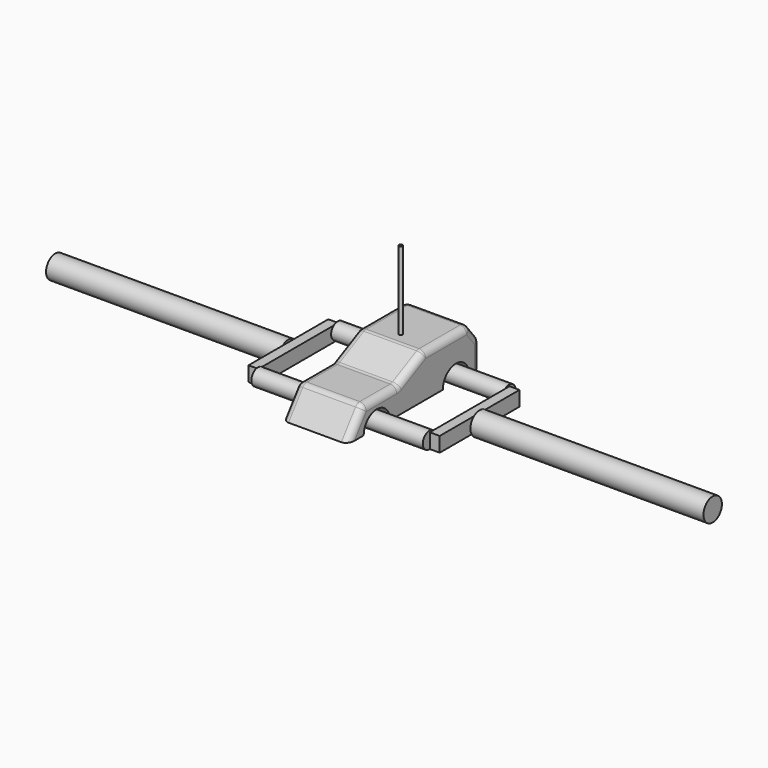
from build123d import *

# Parameters (mm, degrees)
F1_DEPTH  = 25.4
F2_R      = 5.08
F4_DEPTH  = 10.16
F6_DEPTH  = 10.16
F7_R      = 6.35
F8_DEPTH  = 50.8
F10_W     = 76.8076643543
F10_H     = 11.4133090087
F11_DEPTH = 7.62
F13_R     = 8.89
F14_DEPTH = 179.578
F16_R     = 1.27
F17_DEPTH = 60.198


# Not quite as in the source:
# - a feature names something its author has since deleted; it is built from what else it names


with BuildPart() as f1:
    # F0 (on Right) → F1 (new body, symmetric)
    with BuildSketch(Plane.YZ):
        Polygon((-60.8564667081, 20.32), (-76.0964667081, 0), (50.9035332919, 0), (50.9035332919, 20.32), (40.7435332919, 33.02), (-2.4364667081, 33.02), (-27.8364667081, 20.32), align=None)
    extrude(amount=F1_DEPTH, both=True)

    # F2
    f2_edges = [f1.edges().sort_by_distance(p)[0] for p in [
        (25.4, -68.476467, 10.16),
        (25.4, -44.346467, 20.32),
        (25.4, -15.136467, 26.67),
        (25.4, 19.153533, 33.02),
        (25.4, 45.823533, 26.67),
        (25.4, 50.903533, 10.16),
        (0, 50.903533, 20.32),
        (0, 40.743533, 33.02),
        (0, -60.856467, 20.32),
        (0, -27.836467, 20.32),
        (0, -2.436467, 33.02),
        (-25.4, -15.136467, 26.67),
        (-25.4, -44.346467, 20.32),
        (-25.4, -68.476467, 10.16),
        (-25.4, 19.153533, 33.02),
        (-25.4, 50.903533, 10.16),
        (-25.4, 45.823533, 26.67),
    ]]
    fillet(f2_edges, radius=F2_R)

    # F3 (on face) → F4 (cut)
    with BuildSketch(Plane.YZ.offset(25.4)):
        with BuildLine():
            Line((-60.8564667081, 0), (-35.4564667081, 0))
            ThreePointArc((-35.4564667081, 0), (-48.1564667081, 12.7), (-60.8564667081, 0))
        make_face()
        with BuildLine():
            ThreePointArc((40.7435332919, 0), (28.0435332919, 12.7), (15.3435332919, 0))
            Line((15.3435332919, 0), (40.7435332919, 0))
        make_face()
    extrude(amount=-F4_DEPTH, mode=Mode.SUBTRACT)

    # F5 (on face) → F6 (cut)
    with BuildSketch(Plane(origin=(-25.4, 0, 0), x_dir=(0, -1, 0), z_dir=(-1, 0, 0))):
        with BuildLine():
            Line((-40.7435332919, 0), (-15.3435332919, 0))
            ThreePointArc((-15.3435332919, 0), (-28.0435332919, 12.7), (-40.7435332919, 0))
        make_face()
        with BuildLine():
            Line((35.4564667081, 0), (60.8564667081, 0))
            ThreePointArc((60.8564667081, 0), (48.1564667081, 12.7), (35.4564667081, 0))
        make_face()
    extrude(amount=-F6_DEPTH, mode=Mode.SUBTRACT)

    # F7 (on face) → F8 (join)
    with BuildSketch(Plane.YZ.offset(15.24)):
        with BuildLine():
            Line((32.2078052294, 0), (24.5878052294, 0))
            ThreePointArc((24.5878052294, 0), (28.3978052294, -1.27), (32.2078052294, 0))
        make_face()
        with Locations((-48.3666342305, 5.08)):
            Circle(F7_R)
        with BuildLine():
            ThreePointArc((32.2078052294, 0), (34.0774178922, 2.2401936686), (34.7478052294, 5.08))
            ThreePointArc((34.7478052294, 5.08), (25.5579988979, 10.7596126628), (24.5878052294, 0))
            Line((24.5878052294, 0), (32.2078052294, 0))
        make_face()
    extrude(amount=F8_DEPTH)

    # F9: F1 across plane


with BuildPart() as f1_1:
    add(f1.part)
    add(f1.part.mirror(Plane.YZ))

    # F10 (on face) → F11 (join)
    with BuildSketch(Plane.YZ.offset(66.04)):
        with Locations((-9.5459215246, 4.4366544964)):
            Rectangle(F10_W, F10_H)
    extrude(amount=F11_DEPTH)

    # F12: F1 across plane


with BuildPart() as f1_2:
    add(f1_1.part)
    add(f1_1.part.mirror(Plane.YZ))

    # F13 (on face) → F14 (join)
    with BuildSketch(Plane.YZ.offset(73.66)):
        with Locations((-9.5459241474, 3.0935325194)):
            Circle(F13_R)
    extrude(amount=F14_DEPTH)

    # F15: F1 across plane


with BuildPart() as f1_3:
    add(f1_2.part)
    add(f1_2.part.mirror(Plane.YZ))

    # F16 (on face) → F17 (join)
    with BuildSketch(Plane.XY.offset(33.02)):
        with Locations((0, 6.6220072263)):
            Circle(F16_R)
    extrude(amount=F17_DEPTH)


solid = f1_3.part
